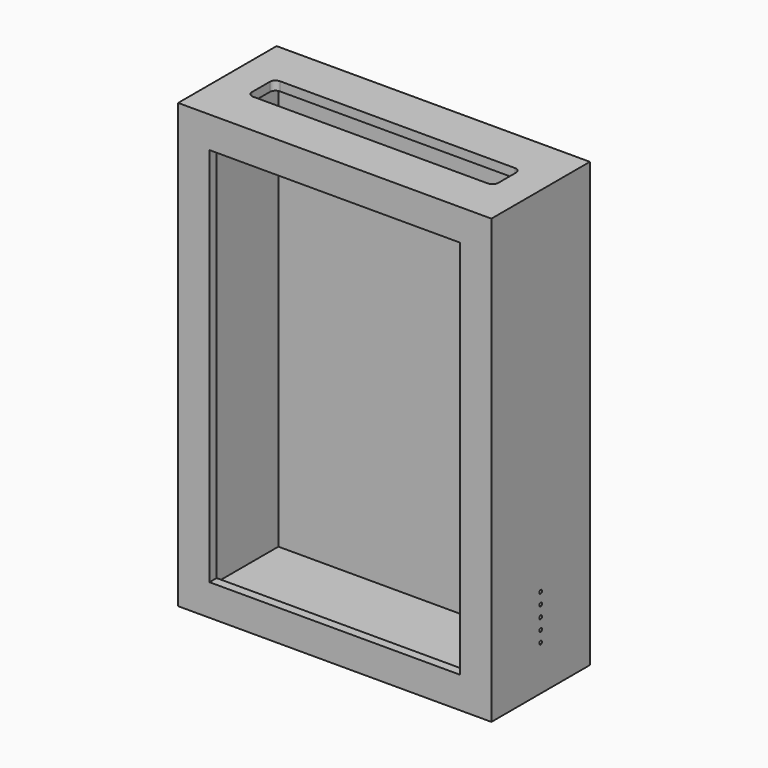
from build123d import *

# Parameters (mm, degrees)
F0_W      = 280
F0_H      = 110
F1_DEPTH  = 8
F2_W      = 280
F2_H      = 110
F2_W_2    = 264
F2_H_2    = 94
F3_DEPTH  = 20
F5_DEPTH  = 340
F6_W      = 224
F6_H      = 8
F7_DEPTH  = 20
F8_W      = 280
F8_H      = 110
F8_W_2    = 264
F8_H_2    = 94
F9_DEPTH  = 8
F10_R     = 1.55
F11_DEPTH = 8
F12_W     = 220
F12_H     = 30
F13_DEPTH = 8
F14_R     = 5


# Not quite as in the source:
# - a feature names something its author has since deleted; it is built from what else it names


with BuildPart() as f1:
    # F0 (on Top) → F1 (new body)
    with BuildSketch(Plane.XY):
        Rectangle(F0_W, F0_H)
    extrude(amount=F1_DEPTH)

    # F2 (on face) → F3 (join)
    with BuildSketch(Plane.XY.offset(8)):
        Rectangle(F2_W, F2_H)
        Rectangle(F2_W_2, F2_H_2, mode=Mode.SUBTRACT)
    extrude(amount=F3_DEPTH)

    # F4 (on face) → F5 (join)
    with BuildSketch(Plane.XY.offset(28)):
        Polygon((-132, -47), (-132, 47), (132, 47), (132, -47), (112, -47), (112, -55), (140, -55), (140, 55), (-140, 55), (-140, -55), (-112, -55), (-112, -47), align=None)
    extrude(amount=F5_DEPTH)

    # F6 (on face) → F7 (join)
    with BuildSketch(Plane.XY.offset(368)):
        Polygon((-112, -47), (-132, -47), (-132, 47), (132, 47), (132, -47), (112, -47), (112, -55), (140, -55), (140, 55), (-140, 55), (-140, -55), (-112, -55), align=None)
        with Locations((0, -51)):
            Rectangle(F6_W, F6_H)
    extrude(amount=F7_DEPTH)

    # F8 (on face) → F9 (join)
    with BuildSketch(Plane.XY.offset(388)):
        Rectangle(F8_W, F8_H)
        Rectangle(F8_W_2, F8_H_2, mode=Mode.SUBTRACT)
        Rectangle(F8_W_2, F8_H_2)
    extrude(amount=F9_DEPTH)

    # F10 (on face) → F11 (cut, through all)
    with BuildSketch(Plane.YZ.offset(140)):
        with Locations((0, 80)):
            Circle(F10_R)
        with Locations((0, 70)):
            Circle(F10_R)
        with Locations((0, 50)):
            Circle(F10_R)
        with Locations((0, 40)):
            Circle(F10_R)
        with Locations((0, 60)):
            Circle(F10_R)
    extrude(amount=-F11_DEPTH, mode=Mode.SUBTRACT)

    # F12 (on face) → F13 (cut, through all)
    with BuildSketch(Plane.XY.offset(396)):
        Rectangle(F12_W, F12_H)
    extrude(amount=-F13_DEPTH, mode=Mode.SUBTRACT)

    # F14
    f14_edges = [f1.edges().sort_by_distance(p)[0] for p in [
        (-110, 15, 392),
        (-110, -15, 392),
        (110, -15, 392),
        (110, 15, 392),
    ]]
    fillet(f14_edges, radius=F14_R)


solid = f1.part
